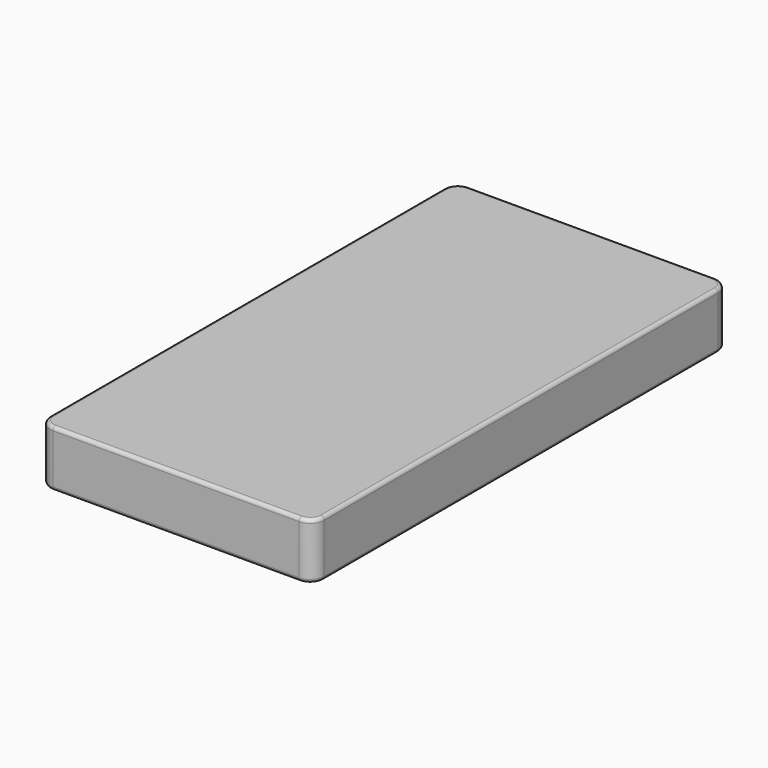
from build123d import *

# Parameters (mm, degrees)
F0_W         = 990.6
F0_H         = 1879.6
F1_DEPTH     = 203.2
F2_R         = 12.7
F3_T1_DEPTH  = 203.2
F3_T4_ANGLE  = 90
F3_T6_ANGLE  = 90
F3_T8_ANGLE  = 90
F3_T10_ANGLE = 90
F3_T12_ANGLE = 90
F3_T14_ANGLE = 90
F3_T16_ANGLE = 90
F3_T18_ANGLE = 90


# Not quite as in the source:
# - a fillet or chamfer that OpenCascade refuses, or shapes differently, is made with other operations: its cross-section is extruded or revolved along the edge and cut away or added


with BuildPart() as f1:
    # F0 (on Top) → F1 (new body)
    with BuildSketch(Plane.XY):
        Rectangle(F0_W, F0_H)
    extrude(amount=F1_DEPTH)

    # F2
    f2_edges = [f1.edges().sort_by_distance(p)[0] for p in [
        (-495.3, 0, 203.2),
        (0, -939.8, 203.2),
        (495.3, 0, 203.2),
        (0, 939.8, 203.2),
        (495.3, 0, 0),
        (0, -939.8, 0),
        (-495.3, 0, 0),
        (0, 939.8, 0),
    ]]
    fillet(f2_edges, radius=F2_R)

    # F3: fillet of radius 50.8 on 4 edges, made by hand

    # F3_s2 → F3_t1 (cut)
    with BuildSketch(Plane.XY):
        with BuildLine():
            ThreePointArc((-495.3, -889), (-480.4210244843, -924.9210244843), (-444.5, -939.8))
            Line((-444.5, -939.8), (-444.5, -940.816))
            Line((-444.5, -940.816), (-496.316, -940.816))
            Line((-496.316, -940.816), (-496.316, -889))
            Line((-496.316, -889), (-495.3, -889))
        make_face()
        with BuildLine():
            ThreePointArc((495.3, -889), (480.4210244843, -924.9210244843), (444.5, -939.8))
            Line((444.5, -939.8), (444.5, -940.816))
            Line((444.5, -940.816), (496.316, -940.816))
            Line((496.316, -940.816), (496.316, -889))
            Line((496.316, -889), (495.3, -889))
        make_face()
        with BuildLine():
            ThreePointArc((444.5, 939.8), (480.4210244843, 924.9210244843), (495.3, 889))
            Line((495.3, 889), (496.316, 889))
            Line((496.316, 889), (496.316, 940.816))
            Line((496.316, 940.816), (444.5, 940.816))
            Line((444.5, 940.816), (444.5, 939.8))
        make_face()
        with BuildLine():
            ThreePointArc((-444.5, 939.8), (-480.4210244843, 924.9210244843), (-495.3, 889))
            Line((-495.3, 889), (-496.316, 889))
            Line((-496.316, 889), (-496.316, 940.816))
            Line((-496.316, 940.816), (-444.5, 940.816))
            Line((-444.5, 940.816), (-444.5, 939.8))
        make_face()
    extrude(amount=F3_T1_DEPTH, mode=Mode.SUBTRACT)

    # F3_s3 → F3_t4 (revolve, cut)
    with BuildSketch(Plane.XZ.offset(-889)):
        with BuildLine():
            ThreePointArc((-482.6, 0), (-491.5802561211, 3.7197438789), (-495.3, 12.7))
            Line((-495.3, 12.7), (-495.3, 0))
            Line((-495.3, 0), (-482.6, 0))
        make_face()
    revolve(axis=Axis((-444.5, 889, 0), (0, 0, -1)), revolution_arc=F3_T4_ANGLE, mode=Mode.SUBTRACT)

    # F3_s5 → F3_t6 (revolve, cut)
    with BuildSketch(Plane.YZ.offset(-444.5)):
        with BuildLine():
            ThreePointArc((927.1, 203.2), (936.0802561211, 199.4802561211), (939.8, 190.5))
            Line((939.8, 190.5), (939.8, 203.2))
            Line((939.8, 203.2), (927.1, 203.2))
        make_face()
    revolve(axis=Axis((-444.5, 889, 203.2), (0, 0, 1)), revolution_arc=F3_T6_ANGLE, mode=Mode.SUBTRACT)

    # F3_s7 → F3_t8 (revolve, cut)
    with BuildSketch(Plane.YZ.offset(444.5)):
        with BuildLine():
            ThreePointArc((927.1, 0), (936.0802561211, 3.7197438789), (939.8, 12.7))
            Line((939.8, 12.7), (939.8, 0))
            Line((939.8, 0), (927.1, 0))
        make_face()
    revolve(axis=Axis((444.5, 889, 0), (0, 0, -1)), revolution_arc=F3_T8_ANGLE, mode=Mode.SUBTRACT)

    # F3_s9 → F3_t10 (revolve, cut)
    with BuildSketch(Plane.XZ.offset(-889)):
        with BuildLine():
            ThreePointArc((482.6, 203.2), (491.5802561211, 199.4802561211), (495.3, 190.5))
            Line((495.3, 190.5), (495.3, 203.2))
            Line((495.3, 203.2), (482.6, 203.2))
        make_face()
    revolve(axis=Axis((444.5, 889, 203.2), (0, 0, 1)), revolution_arc=F3_T10_ANGLE, mode=Mode.SUBTRACT)

    # F3_s11 → F3_t12 (revolve, cut)
    with BuildSketch(Plane.XZ.offset(889)):
        with BuildLine():
            ThreePointArc((482.6, 0), (491.5802561211, 3.7197438789), (495.3, 12.7))
            Line((495.3, 12.7), (495.3, 0))
            Line((495.3, 0), (482.6, 0))
        make_face()
    revolve(axis=Axis((444.5, -889, 0), (0, 0, -1)), revolution_arc=F3_T12_ANGLE, mode=Mode.SUBTRACT)

    # F3_s13 → F3_t14 (revolve, cut)
    with BuildSketch(Plane.YZ.offset(444.5)):
        with BuildLine():
            ThreePointArc((-927.1, 203.2), (-936.0802561211, 199.4802561211), (-939.8, 190.5))
            Line((-939.8, 190.5), (-939.8, 203.2))
            Line((-939.8, 203.2), (-927.1, 203.2))
        make_face()
    revolve(axis=Axis((444.5, -889, 203.2), (0, 0, 1)), revolution_arc=F3_T14_ANGLE, mode=Mode.SUBTRACT)

    # F3_s15 → F3_t16 (revolve, cut)
    with BuildSketch(Plane.YZ.offset(-444.5)):
        with BuildLine():
            ThreePointArc((-927.1, 0), (-936.0802561211, 3.7197438789), (-939.8, 12.7))
            Line((-939.8, 12.7), (-939.8, 0))
            Line((-939.8, 0), (-927.1, 0))
        make_face()
    revolve(axis=Axis((-444.5, -889, 0), (0, 0, -1)), revolution_arc=F3_T16_ANGLE, mode=Mode.SUBTRACT)

    # F3_s17 → F3_t18 (revolve, cut)
    with BuildSketch(Plane.XZ.offset(889)):
        with BuildLine():
            ThreePointArc((-482.6, 203.2), (-491.5802561211, 199.4802561211), (-495.3, 190.5))
            Line((-495.3, 190.5), (-495.3, 203.2))
            Line((-495.3, 203.2), (-482.6, 203.2))
        make_face()
    revolve(axis=Axis((-444.5, -889, 203.2), (0, 0, 1)), revolution_arc=F3_T18_ANGLE, mode=Mode.SUBTRACT)


solid = f1.part
